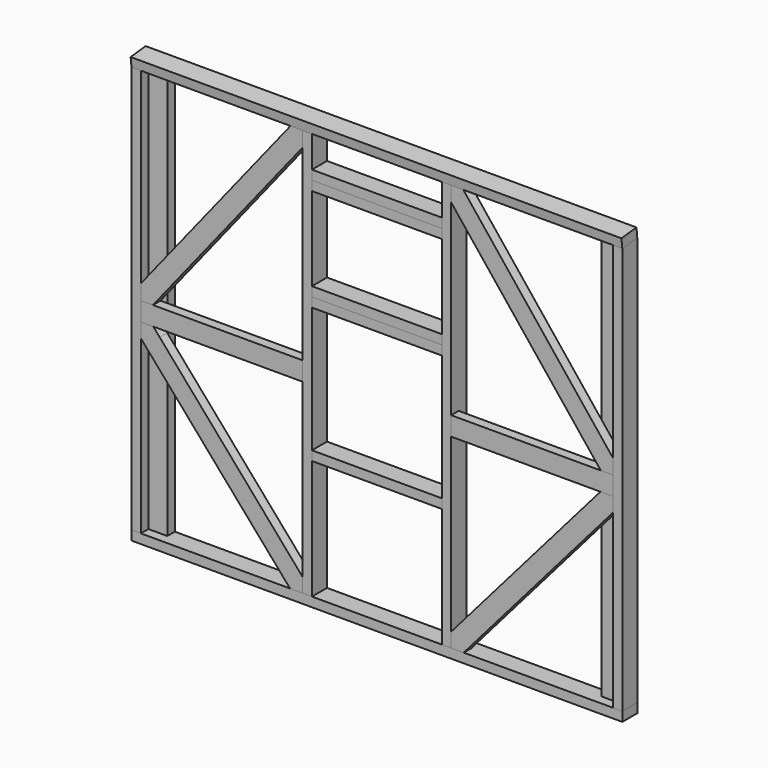
from build123d import *

# Parameters (mm, degrees)
F0_W      = 2344
F0_H      = 90
F1_DEPTH  = 45
F2_W      = 90
F2_H      = 1945.34335
F5_DEPTH  = 45
F4_W      = 90
F4_H      = 1945.34335
F7_DEPTH  = 45
F8_W      = 45
F8_H      = 90
F8_W_2    = 2299
F9_DEPTH  = 45
F10_W     = 620
F10_H     = 45
F11_DEPTH = 90
F12_DEPTH = 90
F13_DEPTH = 45
F10_W_2   = 682
F10_H_2   = 90
F14_DEPTH = 45
F16_START = -45
F16_DEPTH = 45


# Not quite as in the source:
# - a feature names something its author has since deleted; it is built from what else it names


with BuildPart() as f1:
    # F0 (on Top) → F1 (new body)
    with BuildSketch(Plane.XY):
        Rectangle(F0_W, F0_H)
    extrude(amount=F1_DEPTH)


with BuildPart() as f5:
    # F2 (on face) → F5 (new body)
    with BuildSketch(Plane(origin=(-1172, 0, 0), x_dir=(0, -1, 0), z_dir=(-1, 0, 0))):
        with Locations((0, 1017.671675)):
            Rectangle(F2_W, F2_H)
        Polygon((-45, 2000), (-45, 1990.34335), (45, 1990.34335), align=None)
    extrude(amount=-F5_DEPTH)


with BuildPart() as f6_1:
    # F6: instance of F5
    add(f5.part.mirror(Plane.YZ))


with BuildPart() as f7:
    # F4 (on offset) → F7 (new body)
    with BuildSketch(Plane.YZ.offset(-310)):
        Polygon((-45, 1990.34335), (45, 1990.34335), (45, 2000), align=None)
        with Locations((0, 1017.671675)):
            Rectangle(F4_W, F4_H)
    extrude(amount=-F7_DEPTH)


with BuildPart() as f9:
    # F8 (on face) → F9 (new body)
    with BuildSketch(Plane(origin=(0, -211.6376922213, 1972.4637736601), x_dir=(1, 0, 0), z_dir=(0, -0.1066837724, 0.9942930014))):
        with Locations((-1149.5, 212.5941518041)):
            Rectangle(F8_W, F8_H)
        with Locations((22.5, 212.5941518041)):
            Rectangle(F8_W_2, F8_H)
    extrude(amount=F9_DEPTH)


with BuildPart() as f11:
    # F10 (on face) → F11 (new body)
    with BuildSketch(Plane.XZ.offset(45)):
        with Locations((0, 1282.5)):
            Rectangle(F10_W, F10_H)
    extrude(amount=-F11_DEPTH)


with BuildPart() as f11b:
    # F10 (on face) → F11, piece 2 (new body)
    with BuildSketch(Plane.XZ.offset(45)):
        with Locations((0, 1772.5)):
            Rectangle(F10_W, F10_H)
    extrude(amount=-F11_DEPTH)


with BuildPart() as f12:
    # F10 (on face) → F12 (new body)
    with BuildSketch(Plane.XZ.offset(45)):
        with Locations((0, 637.5)):
            Rectangle(F10_W, F10_H)
    extrude(amount=-F12_DEPTH)


with BuildPart() as f12b:
    # F10 (on face) → F12, piece 2 (new body)
    with BuildSketch(Plane.XZ.offset(45)):
        with Locations((0, 1327.5)):
            Rectangle(F10_W, F10_H)
    extrude(amount=-F12_DEPTH)


with BuildPart() as f12c:
    # F10 (on face) → F12, piece 3 (new body)
    with BuildSketch(Plane.XZ.offset(45)):
        with Locations((0, 1817.5)):
            Rectangle(F10_W, F10_H)
    extrude(amount=-F12_DEPTH)


with BuildPart() as f13:
    # F10 (on face) → F13 (new body)
    with BuildSketch(Plane.XZ.offset(45)):
        Polygon((-355, 1918.2352214167), (-355, 1990.34335), (-412.5908448117, 1990.34335), (-1037, 1208.5354810911), (-1037, 1064.3192239245), align=None)
        Polygon((-1037, 1064.3192239245), (-1037, 1208.5354810911), (-1127, 1095.8486192519), (-1127, 1023.7404906686), (-1069.4091551883, 1023.7404906686), align=None)
    extrude(amount=-F13_DEPTH)


with BuildPart() as f13b:
    # F10 (on face) → F13, piece 2 (new body)
    with BuildSketch(Plane.XZ.offset(45)):
        Polygon((-355, 45), (-355, 113.6202558639), (-1037, 898.751103838), (-1037, 761.5105921102), (-414.6066434275, 45), align=None)
        Polygon((-1067.3933565725, 933.7404906686), (-1127, 933.7404906686), (-1127, 865.1202348048), (-1037, 761.5105921102), (-1037, 898.751103838), align=None)
    extrude(amount=-F13_DEPTH)


with BuildPart() as f14:
    # F10 (on face) → F14 (new body)
    with BuildSketch(Plane.XZ.offset(45)):
        Polygon((-1037, 933.7404906686), (-1037, 1023.7404906686), (-1069.4091551883, 1023.7404906686), (-1127, 1023.7404906686), (-1127, 933.7404906686), (-1067.3933565725, 933.7404906686), align=None)
        with Locations((-696, 978.7404906686)):
            Rectangle(F10_W_2, F10_H_2)
    extrude(amount=-F14_DEPTH)


with BuildPart() as f15_1:
    # F15: instance of F13
    add(f13.part.mirror(Plane.YZ))


with BuildPart() as f15_2:
    # F15: instance of F13b
    add(f13b.part.mirror(Plane.YZ))


with BuildPart() as f15_3:
    # F15: instance of F7
    add(f7.part.mirror(Plane.YZ))


with BuildPart() as f15_4:
    # F15: instance of F14
    add(f14.part.mirror(Plane.YZ))


with BuildPart() as f16:
    # F10 (on face) → F16 (new body)
    with BuildSketch(Plane.XZ.offset(45).offset(F16_START)):
        Polygon((-1127, 1095.8486192519), (-1037, 1208.5354810911), (-1037, 1990.34335), (-1127, 1990.34335), align=None)
        Polygon((-1037, 1064.3192239245), (-1037, 1208.5354810911), (-1127, 1095.8486192519), (-1127, 1023.7404906686), (-1069.4091551883, 1023.7404906686), align=None)
        Polygon((-1037, 1023.7404906686), (-1037, 1064.3192239245), (-1069.4091551883, 1023.7404906686), align=None)
        Polygon((-1037, 933.7404906686), (-1037, 1023.7404906686), (-1069.4091551883, 1023.7404906686), (-1127, 1023.7404906686), (-1127, 933.7404906686), (-1067.3933565725, 933.7404906686), align=None)
        Polygon((-1037, 898.751103838), (-1037, 933.7404906686), (-1067.3933565725, 933.7404906686), align=None)
        Polygon((-1067.3933565725, 933.7404906686), (-1127, 933.7404906686), (-1127, 865.1202348048), (-1037, 761.5105921102), (-1037, 898.751103838), align=None)
        Polygon((-1037, 761.5105921102), (-1127, 865.1202348048), (-1127, 45), (-1037, 45), align=None)
    extrude(amount=-F16_DEPTH)


with BuildPart() as f17_1:
    # F17: instance of F16
    add(f16.part.mirror(Plane.YZ))


solid = Compound([f1.part, f5.part, f6_1.part, f7.part, f9.part, f11.part, f11b.part, f12.part, f12b.part, f12c.part, f13.part, f13b.part, f14.part, f15_1.part, f15_2.part, f15_3.part, f15_4.part, f16.part, f17_1.part])
